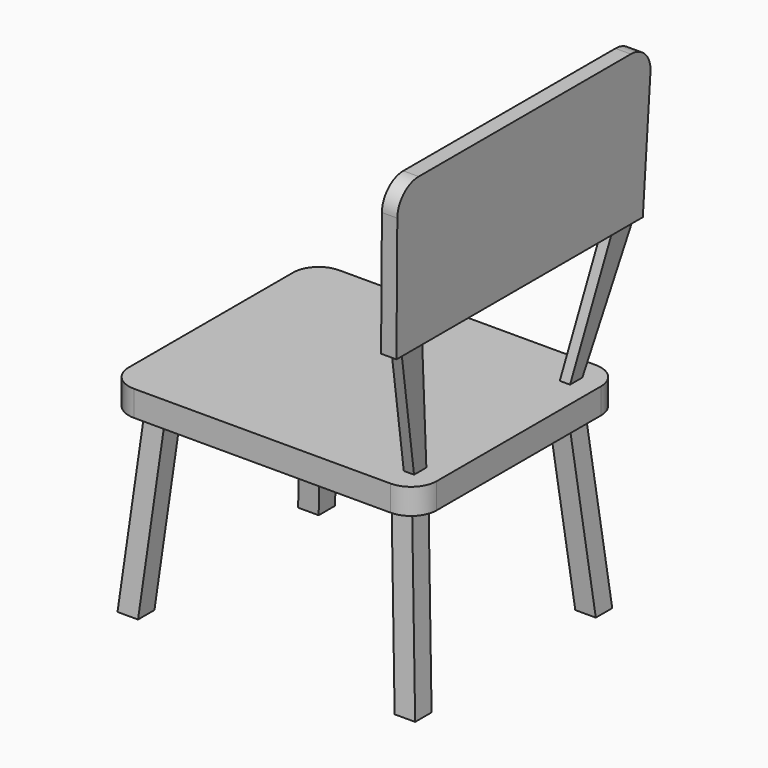
from build123d import *

# Parameters (mm, degrees)
F1_DEPTH = 5
F2_W     = 4
F2_H     = 4
F4_W     = 4
F4_H     = 4
F7_W     = 2
F7_H     = 3
F9_W     = 2
F9_H     = 5
F11_W    = 3
F11_H    = 30
F13_W    = 3
F13_H    = 31
F16_R    = 5


with BuildPart() as f1:
    # F0 (on Top) → F1 (new body)
    with BuildSketch(Plane.XY):
        with BuildLine():
            Line((-30, 0), (0, 0))
            Line((0, 0), (0, 25))
            Line((0, 25), (-25, 25))
            ThreePointArc((-25, 25), (-28.5355339059, 23.5355339059), (-30, 20))
            Line((-30, 20), (-30, 0))
        make_face()
    extrude(amount=F1_DEPTH)

    # F2 (on face) → F5 section 0
    with BuildSketch(Plane(origin=(0, 0, 0), x_dir=(1, 0, 0), z_dir=(0, 0, -1))):
        with Locations((-24, -19)):
            Rectangle(F2_W, F2_H)
    # F4 (on offset) → F5 section 1
    with BuildSketch(Plane(origin=(0, 0, -35), x_dir=(1, 0, 0), z_dir=(0, 0, -1))):
        with Locations((-27, -22)):
            Rectangle(F4_W, F4_H)
    loft()

    # F6: F1 across plane


with BuildPart() as f1_1:
    add(f1.part)
    add(f1.part.mirror(Plane.YZ))

    # F7 (on face) → F10 section 0
    with BuildSketch(Plane.XY.offset(5)):
        with Locations((24.9823927879, 19)):
            Rectangle(F7_W, F7_H)
    # F9 (on offset) → F10 section 1
    with BuildSketch(Plane.XY.offset(30)):
        with Locations((28.6593784243, 25.6122151948)):
            Rectangle(F9_W, F9_H)
    loft()

    # F11 (on offset) → F14 section 0
    with BuildSketch(Plane.XY.offset(30)):
        with Locations((28.6593784243, 15)):
            Rectangle(F11_W, F11_H)
    # F13 (on offset) → F14 section 1
    with BuildSketch(Plane.XY.offset(60)):
        with Locations((29.6593784243, 15.5)):
            Rectangle(F13_W, F13_H)
    loft()

    # F15: F1 across plane


with BuildPart() as f1_2:
    add(f1_1.part)
    add(f1_1.part.mirror(Plane.XZ))

    # F16
    f16_edges = [f1_2.edges().sort_by_distance(p)[0] for p in [
        (29.659378, 31, 60),
        (29.659378, -31, 60),
    ]]
    fillet(f16_edges, radius=F16_R)

    # F17: F1 across plane


with BuildPart() as f1_3:
    add(f1_2.part)
    add(f1_2.part.mirror(Plane.XZ))


solid = f1_3.part
